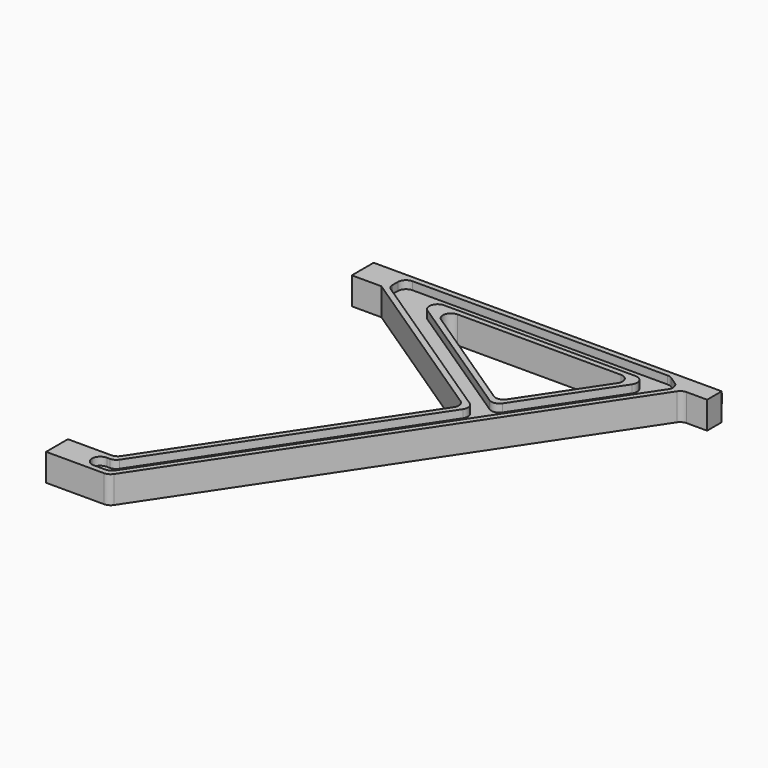
from build123d import *

# Parameters (mm, degrees)
F1_DEPTH    = 1.5875
F0_W        = 3.175
F0_H        = 3.81
F2_DEPTH    = 3.81
F0_H_2      = 3.175
F3_DEPTH    = 1.5875
F5_R        = 2.28599
F6_C1_SIZE2 = 0.254
F6_C1_SIZE  = 0.762
F6_C2_SIZE2 = 0.254
F6_C2_SIZE  = 0.762
F6_C3_SIZE2 = 0.762
F6_C3_SIZE  = 0.254
F6_C4_SIZE2 = 0.762
F6_C4_SIZE  = 0.254


# Not quite as in the source:
# - a fillet or chamfer is up to 0.001 mm smaller than in the source, because OpenCascade refuses the exact size


with BuildPart() as f1:
    # F0 (on Top) → F1 (new body, symmetric)
    with BuildSketch(Plane.XY):
        Polygon((84.7879795397, 75.6059451024), (107.4843514416, 109.6505029552), (102.7961058745, 112.776), (28.5815359464, 112.776), (28.5815359464, 107.4966776252), (78.4441827097, 74.332540073), (32.9531559943, 6.096), (28.5815359464, 6.096), (28.5815359464, 1.524), (35.4000161381, 1.524), (82.2518902426, 71.8018111567), align=None)
        Polygon((35.7737204145, 108.204), (101.0251559943, 108.204), (80.9802734819, 78.1366762315), align=None, mode=Mode.SUBTRACT)
    extrude(amount=F1_DEPTH, both=True)

    # F0 (on Top) → F2 (join, symmetric)
    with BuildSketch(Plane.XY):
        Polygon((27.0575359464, 3.81), (27.0575359464, 0), (36.215636186, 0), (109.0289695194, 109.22), (115.9575359464, 109.22), (115.9575359464, 114.3), (113.7350359464, 114.3), (110.5600359464, 114.3), (103.2575359464, 114.3), (27.0575359464, 114.3), (18.8025359464, 114.3), (18.8025359464, 106.68), (23.8825359464, 106.68), (23.8825359464, 110.49), (27.0575359464, 110.49), (27.0575359464, 106.68), (76.2944590233, 73.8553846154), (32.1375359464, 7.62), (27.0575359464, 7.62), (18.8025359464, 7.62), (18.8025359464, 0), (23.8825359464, 0), (23.8825359464, 3.81), align=None)
        Polygon((102.7961058745, 112.776), (107.4843514416, 109.6505029552), (84.7879795397, 75.6059451024), (82.2518902426, 71.8018111567), (35.4000161381, 1.524), (28.5815359464, 1.524), (28.5815359464, 6.096), (32.9531559943, 6.096), (78.4441827097, 74.332540073), (28.5815359464, 107.4966776252), (28.5815359464, 112.776), align=None, mode=Mode.SUBTRACT)
        Polygon((80.9802734819, 78.1366762315), (101.0251559943, 108.204), (35.7737204145, 108.204), align=None)
        Polygon((80.5212745185, 80.1956078582), (40.7946863059, 106.68), (98.1775359464, 106.68), align=None, mode=Mode.SUBTRACT)
        with Locations((25.4700359464, 1.905)):
            Rectangle(F0_W, F0_H)
        with Locations((25.4700359464, 108.585)):
            Rectangle(F0_W, F0_H)
    extrude(amount=F2_DEPTH, both=True)

    # F0 (on Top) → F3 (join, symmetric)
    with BuildSketch(Plane.XY):
        with Locations((112.1475359464, 115.8875)):
            Rectangle(F0_W, F0_H_2)
    extrude(amount=F3_DEPTH, both=True)


with BuildPart() as f1_1:
    # F4: moved
    add(f1.part.moved(Location((0, 0, 3.81))))

    # F5 (radius 2.286 in the source; OpenCascade refuses exactly that, so slightly less here)
    f5_edges = [f1_1.edges().sort_by_distance(p)[0] for p in [
        (35.77372, 108.204, 6.50875),
        (35.77372, 108.204, 1.11125),
        (101.025156, 108.204, 6.50875),
        (101.025156, 108.204, 1.11125),
        (80.980273, 78.136676, 1.11125),
        (80.980273, 78.136676, 6.50875),
        (78.444183, 74.33254, 6.50875),
        (78.444183, 74.33254, 1.11125),
        (102.796106, 112.776, 6.50875),
        (102.796106, 112.776, 1.11125),
        (28.581536, 112.776, 6.50875),
        (28.581536, 107.496678, 6.50875),
        (28.581536, 107.496678, 1.11125),
        (28.581536, 112.776, 1.11125),
        (32.953156, 6.096, 6.50875),
        (32.953156, 6.096, 1.11125),
        (35.400016, 1.524, 1.11125),
        (35.400016, 1.524, 6.50875),
        (28.581536, 6.096, 6.50875),
        (28.581536, 1.524, 6.50875),
        (28.581536, 1.524, 1.11125),
        (28.581536, 6.096, 1.11125),
        (107.484351, 109.650503, 6.50875),
        (107.484351, 109.650503, 1.11125),
        (109.02897, 109.22, 3.81),
        (36.215636, 0, 3.81),
        (76.294459, 73.855385, 3.81),
        (32.137536, 7.62, 3.81),
        (40.794686, 106.68, 3.81),
        (80.521275, 80.195608, 3.81),
        (98.177536, 106.68, 3.81),
    ]]
    fillet(f5_edges, radius=F5_R)

    # F6: chamfer of 0.254 x 0.762 on 4 edges, made by hand

    # F6_c1
    f6_c1_edges = [f1_1.edges().sort_by_distance(p)[0] for p in [
        (110.5600359464, 117.475, 3.81),
    ]]
    f6_c1_side = f1_1.faces().sort_by_distance((110.5600359464, 117.46992, 3.81))[0]
    chamfer(f6_c1_edges, length=F6_C1_SIZE, length2=F6_C1_SIZE2, reference=f6_c1_side)

    # F6_c2
    f6_c2_edges = [f1_1.edges().sort_by_distance(p)[0] for p in [
        (112.2745359464, 117.475, 5.3975),
    ]]
    f6_c2_side = f1_1.faces().sort_by_distance((112.2745359464, 117.46992, 5.3975))[0]
    chamfer(f6_c2_edges, length=F6_C2_SIZE, length2=F6_C2_SIZE2, reference=f6_c2_side)

    # F6_c3
    f6_c3_edges = [f1_1.edges().sort_by_distance(p)[0] for p in [
        (113.7350359464, 117.475, 3.683),
    ]]
    f6_c3_side = f1_1.faces().sort_by_distance((113.7299559464, 117.475, 3.683))[0]
    chamfer(f6_c3_edges, length=F6_C3_SIZE, length2=F6_C3_SIZE2, reference=f6_c3_side)

    # F6_c4
    f6_c4_edges = [f1_1.edges().sort_by_distance(p)[0] for p in [
        (112.1475359464, 117.475, 2.2225),
    ]]
    f6_c4_side = f1_1.faces().sort_by_distance((112.1475359464, 117.475, 2.22758))[0]
    chamfer(f6_c4_edges, length=F6_C4_SIZE, length2=F6_C4_SIZE2, reference=f6_c4_side)


solid = f1_1.part
